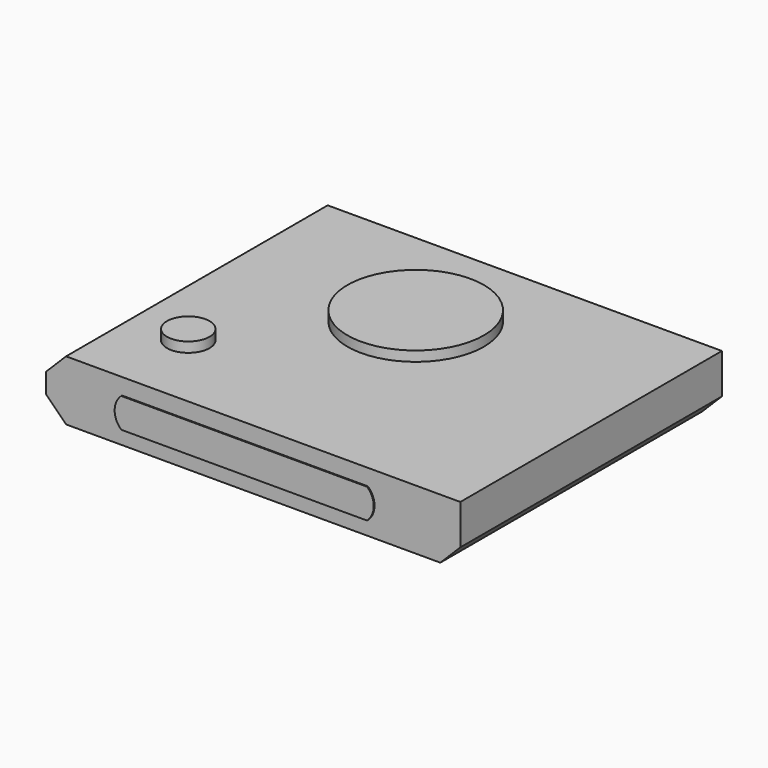
from build123d import *

# Parameters (mm, degrees)
F0_W         = 105.2784845233
F0_H         = 83.1132326275
F1_DEPTH     = 15.24
F2_SIZE      = 5.08
F3_SIZE      = 5.08
F4_R         = 17.3387510066
F4_R_2       = 5.4081350991
F5_DEPTH     = 2.54
F6_W         = 68.5574207455
F6_H         = 7.6610487886
F7_DEPTH     = 0.254
F8_W         = 72.6598203182
F8_H         = 7.5589888729
F9_DEPTH     = 0.254
F10_T1_DEPTH = 13.3181495789
F11_R        = 5.08
F12_T1_DEPTH = 13.3181495789
F13_R        = 5.08


# Not quite as in the source:
# - a fillet or chamfer that OpenCascade refuses, or shapes differently, is made with other operations: its cross-section is extruded or revolved along the edge and cut away or added


with BuildPart() as f1:
    # F0 (on Top) → F1 (new body)
    with BuildSketch(Plane.XY):
        with Locations((16.9621892273, -13.4625034407)):
            Rectangle(F0_W, F0_H)
    extrude(amount=F1_DEPTH)

    # F2
    f2_edges = [f1.edges().sort_by_distance(p)[0] for p in [
        (-35.677053, -13.462503, 15.24),
        (-35.677053, -13.462503, 0),
    ]]
    chamfer(f2_edges, length=F2_SIZE)

    # F3
    f3_edges = [f1.edges().sort_by_distance(p)[0] for p in [
        (69.601431, -13.462503, 0),
    ]]
    chamfer(f3_edges, length=F3_SIZE)

    # F4 (on face) → F5 (join)
    with BuildSketch(Plane.XY.offset(15.24)):
        with Locations((14.2443789936, 0)):
            Circle(F4_R)
        with Locations((-15.9631352872, -34.4845345244)):
            Circle(F4_R_2)
    extrude(amount=F5_DEPTH)

    # F6 (on face) → F7 (join)
    with BuildSketch(Plane(origin=(0, 28.0941128731, 0), x_dir=(-1, 0, 0), z_dir=(0, 1, 0))):
        with Locations((-17.0010654256, 7.0315066259)):
            Rectangle(F6_W, F6_H)
    extrude(amount=F7_DEPTH)

    # F8 (on face) → F9 (join)
    with BuildSketch(Plane.XZ.offset(55.0191197544)):
        with Locations((14.8761942983, 7.3211907875)):
            Rectangle(F8_W, F8_H)
    extrude(amount=F9_DEPTH)

    # F10: chamfer of 5.08 on 4 edges, made by hand

    # F10_s2 → F10_t1 (cut)
    with BuildSketch(Plane.XZ.offset(55.0191197544)):
        Polygon((51.2061044574, 8.621696351), (46.1261044574, 3.541696351), (51.2061044574, 3.541696351), align=None)
        Polygon((51.2061044574, 6.0206852239), (46.1261044574, 11.1006852239), (51.2061044574, 11.1006852239), align=None)
        Polygon((-21.4537158608, 6.0206852239), (-16.3737158608, 11.1006852239), (-21.4537158608, 11.1006852239), align=None)
        Polygon((-16.3737158608, 3.541696351), (-21.4537158608, 8.621696351), (-21.4537158608, 3.541696351), align=None)
    extrude(amount=F10_T1_DEPTH, mode=Mode.SUBTRACT)

    # F11
    f11_edges = [f1.edges().sort_by_distance(p)[0] for p in [
        (-20.15321, -55.14612, 7.321191),
        (49.905599, -55.14612, 7.321191),
    ]]
    fillet(f11_edges, radius=F11_R)

    # F12: chamfer of 5.08 on 4 edges, made by hand

    # F12_s2 → F12_t1 (cut)
    with BuildSketch(Plane.XZ.offset(-41.4122624519)):
        Polygon((51.2797757983, 5.7820310202), (46.1997757983, 10.8620310202), (51.2797757983, 10.8620310202), align=None)
        Polygon((46.1997757983, 3.2009822316), (51.2797757983, 8.2809822316), (51.2797757983, 3.2009822316), align=None)
        Polygon((-17.2776449472, 8.2809822316), (-12.1976449472, 3.2009822316), (-17.2776449472, 3.2009822316), align=None)
        Polygon((-17.2776449472, 5.7820310202), (-12.1976449472, 10.8620310202), (-17.2776449472, 10.8620310202), align=None)
    extrude(amount=F12_T1_DEPTH, mode=Mode.SUBTRACT)

    # F13
    f13_edges = [f1.edges().sort_by_distance(p)[0] for p in [
        (-16.028169, 28.221113, 7.031507),
        (50.0303, 28.221113, 7.031507),
    ]]
    fillet(f13_edges, radius=F13_R)


solid = f1.part
